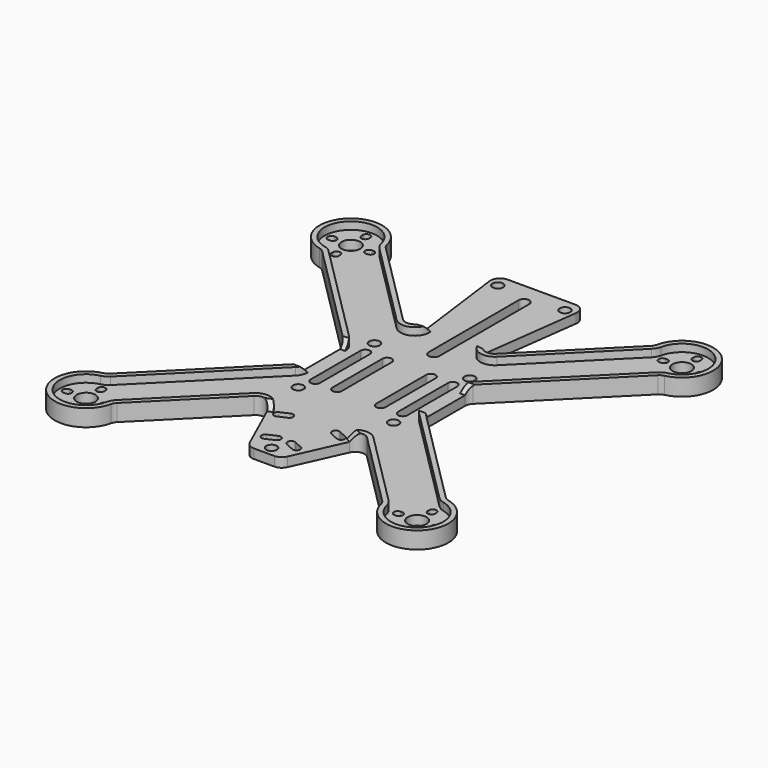
from build123d import *

# Parameters (mm, degrees)
F0_R     = 3
F0_R_2   = 1.7
F1_DEPTH = 3
F2_DEPTH = 5.4
F3_SIZE  = 2.39999


# Not quite as in the source:
# - a fillet or chamfer is up to 0.001 mm smaller than in the source, because OpenCascade refuses the exact size


with BuildPart() as f1:
    # F0 (on Top) → F1 (new body)
    with BuildSketch(Plane.XY):
        with BuildLine():
            Line((20, 0), (20, 7.4436508139))
            Line((20, 7.4436508139), (18.4, 7.4436508139))
            ThreePointArc((18.4, 7.4436508139), (18.7501541504, 9.2039946028), (19.7473088065, 10.6963420074))
            Line((19.7473088065, 10.6963420074), (52.626503914, 43.5755371148))
            ThreePointArc((52.626503914, 43.5755371148), (53.6562447149, 44.3500647573), (54.8604029925, 44.8086081338))
            ThreePointArc((54.8604029925, 44.8086081338), (58.939696962, 58.939696962), (44.8086081338, 54.8604029925))
            ThreePointArc((44.8086081338, 54.8604029925), (44.3500647573, 53.6562447149), (43.5755371148, 52.626503914))
            Line((43.5755371148, 52.626503914), (16.0551666535, 25.1061334527))
            ThreePointArc((16.0551666535, 25.1061334527), (10.770303635, 24.2320489467), (8.241146365, 28.9540362775))
            Line((8.241146365, 28.9540362775), (9.8276956154, 28.7470061448))
            Line((9.8276956154, 28.7470061448), (13.8552706772, 59.6118185013))
            ThreePointArc((13.8552706772, 59.6118185013), (13.1348803837, 61.9793250749), (10.8804908326, 63))
            Line((10.8804908326, 63), (0, 63))
            Line((0, 63), (-10.8804908326, 63))
            ThreePointArc((-10.8804908326, 63), (-13.1348803837, 61.9793250749), (-13.8552706772, 59.6118185013))
            Line((-13.8552706772, 59.6118185013), (-9.8276956154, 28.7470061448))
            Line((-9.8276956154, 28.7470061448), (-8.241146365, 28.9540362775))
            ThreePointArc((-8.241146365, 28.9540362775), (-10.770303635, 24.2320489467), (-16.0551666535, 25.1061334527))
            Line((-16.0551666535, 25.1061334527), (-43.5755371148, 52.626503914))
            ThreePointArc((-43.5755371148, 52.626503914), (-44.3500647573, 53.6562447149), (-44.8086081338, 54.8604029925))
            ThreePointArc((-44.8086081338, 54.8604029925), (-58.939696962, 58.939696962), (-54.8604029925, 44.8086081338))
            ThreePointArc((-54.8604029925, 44.8086081338), (-53.6562447149, 44.3500647573), (-52.626503914, 43.5755371148))
            Line((-52.626503914, 43.5755371148), (-19.7473088065, 10.6963420074))
            ThreePointArc((-19.7473088065, 10.6963420074), (-18.7501541504, 9.2039946028), (-18.4, 7.4436508139))
            Line((-18.4, 7.4436508139), (-20, 7.4436508139))
            Line((-20, 7.4436508139), (-20, 0))
            Line((-20, 0), (-20, -7.4436508139))
            Line((-20, -7.4436508139), (-18.4, -7.4436508139))
            ThreePointArc((-18.4, -7.4436508139), (-18.7501541504, -9.2039946028), (-19.7473088065, -10.6963420074))
            Line((-19.7473088065, -10.6963420074), (-52.626503914, -43.5755371148))
            ThreePointArc((-52.626503914, -43.5755371148), (-53.6562447149, -44.3500647573), (-54.8604029925, -44.8086081338))
            ThreePointArc((-54.8604029925, -44.8086081338), (-58.939696962, -58.939696962), (-44.8086081338, -54.8604029925))
            ThreePointArc((-44.8086081338, -54.8604029925), (-44.3500647573, -53.6562447149), (-43.5755371148, -52.626503914))
            Line((-43.5755371148, -52.626503914), (-19.2033018184, -28.2542686176))
            ThreePointArc((-19.2033018184, -28.2542686176), (-15.1223546276, -26.9821402563), (-11.7566370429, -29.6173604901))
            Line((-11.7566370429, -29.6173604901), (-13.2154104627, -30.2746124278))
            Line((-13.2154104627, -30.2746124278), (-6.025635767, -46.2323473832))
            ThreePointArc((-6.025635767, -46.2323473832), (-4.9187718494, -47.5196271698), (-3.2904356048, -48))
            Line((-3.2904356048, -48), (0, -48))
            Line((0, -48), (3.2904356048, -48))
            ThreePointArc((3.2904356048, -48), (4.9187718494, -47.5196271698), (6.025635767, -46.2323473832))
            Line((6.025635767, -46.2323473832), (13.2154104627, -30.2746124278))
            Line((13.2154104627, -30.2746124278), (11.7566370429, -29.6173604901))
            ThreePointArc((11.7566370429, -29.6173604901), (15.1223546276, -26.9821402563), (19.2033018184, -28.2542686176))
            Line((19.2033018184, -28.2542686176), (43.5755371148, -52.626503914))
            ThreePointArc((43.5755371148, -52.626503914), (44.3500647573, -53.6562447149), (44.8086081338, -54.8604029925))
            ThreePointArc((44.8086081338, -54.8604029925), (58.939696962, -58.939696962), (54.8604029925, -44.8086081338))
            ThreePointArc((54.8604029925, -44.8086081338), (53.6562447149, -44.3500647573), (52.626503914, -43.5755371148))
            Line((52.626503914, -43.5755371148), (19.7473088065, -10.6963420074))
            ThreePointArc((19.7473088065, -10.6963420074), (18.7501541504, -9.2039946028), (18.4, -7.4436508139))
            Line((18.4, -7.4436508139), (20, -7.4436508139))
            Line((20, -7.4436508139), (20, 0))
        make_face()
        with BuildLine():
            Line((-54.2, -59.25), (-54.2, -58.75))
            ThreePointArc((-54.2, -58.75), (-53, -57.55), (-51.8, -58.75))
            Line((-51.8, -58.75), (-51.8, -59.25))
            ThreePointArc((-51.8, -59.25), (-53, -60.45), (-54.2, -59.25))
        make_face(mode=Mode.SUBTRACT)
        with BuildLine():
            Line((-59.25, -51.8), (-58.75, -51.8))
            ThreePointArc((-58.75, -51.8), (-57.55, -53), (-58.75, -54.2))
            Line((-58.75, -54.2), (-59.25, -54.2))
            ThreePointArc((-59.25, -54.2), (-60.45, -53), (-59.25, -51.8))
        make_face(mode=Mode.SUBTRACT)
        with Locations((-53, -53)):
            Circle(F0_R, mode=Mode.SUBTRACT)
        with BuildLine():
            Line((-46.75, -54.2), (-47.25, -54.2))
            ThreePointArc((-47.25, -54.2), (-48.45, -53), (-47.25, -51.8))
            Line((-47.25, -51.8), (-46.75, -51.8))
            ThreePointArc((-46.75, -51.8), (-45.55, -53), (-46.75, -54.2))
        make_face(mode=Mode.SUBTRACT)
        with BuildLine():
            Line((-51.8, -46.75), (-51.8, -47.25))
            ThreePointArc((-51.8, -47.25), (-53, -48.45), (-54.2, -47.25))
            Line((-54.2, -47.25), (-54.2, -46.75))
            ThreePointArc((-54.2, -46.75), (-53, -45.55), (-51.8, -46.75))
        make_face(mode=Mode.SUBTRACT)
        with BuildLine():
            ThreePointArc((-4.4950166018, -42.3264274481), (-6.0820356199, -41.7252863365), (-5.4808945083, -40.1382673183))
            Line((-5.4808945083, -40.1382673183), (-2.7456943461, -38.9059199351))
            ThreePointArc((-2.7456943461, -38.9059199351), (-1.158675328, -39.5070610467), (-1.7598164396, -41.0940800649))
            Line((-1.7598164396, -41.0940800649), (-4.4950166018, -42.3264274481))
        make_face(mode=Mode.SUBTRACT)
        with BuildLine():
            ThreePointArc((-9.629797365, -30.9297601057), (-11.2168163832, -30.3286189941), (-10.6156752716, -28.7415999759))
            Line((-10.6156752716, -28.7415999759), (-7.8804751094, -27.5092525927))
            ThreePointArc((-7.8804751094, -27.5092525927), (-6.2934560912, -28.1103937043), (-6.8945972028, -29.6974127225))
            Line((-6.8945972028, -29.6974127225), (-9.629797365, -30.9297601057))
        make_face(mode=Mode.SUBTRACT)
        with Locations((-15.25, -15.25)):
            Circle(F0_R_2, mode=Mode.SUBTRACT)
        with Locations((0, -45)):
            Circle(F0_R_2, mode=Mode.SUBTRACT)
        with BuildLine():
            Line((2.7456943461, -38.9059199351), (5.4808945083, -40.1382673183))
            ThreePointArc((5.4808945083, -40.1382673183), (6.0820356199, -41.7252863365), (4.4950166018, -42.3264274481))
            Line((4.4950166018, -42.3264274481), (1.7598164396, -41.0940800649))
            ThreePointArc((1.7598164396, -41.0940800649), (1.158675328, -39.5070610467), (2.7456943461, -38.9059199351))
        make_face(mode=Mode.SUBTRACT)
        with BuildLine():
            ThreePointArc((47.25, -51.8), (48.45, -53), (47.25, -54.2))
            Line((47.25, -54.2), (46.75, -54.2))
            ThreePointArc((46.75, -54.2), (45.55, -53), (46.75, -51.8))
            Line((46.75, -51.8), (47.25, -51.8))
        make_face(mode=Mode.SUBTRACT)
        with BuildLine():
            ThreePointArc((54.2, -59.25), (53, -60.45), (51.8, -59.25))
            Line((51.8, -59.25), (51.8, -58.75))
            ThreePointArc((51.8, -58.75), (53, -57.55), (54.2, -58.75))
            Line((54.2, -58.75), (54.2, -59.25))
        make_face(mode=Mode.SUBTRACT)
        with Locations((53, -53)):
            Circle(F0_R, mode=Mode.SUBTRACT)
        with BuildLine():
            ThreePointArc((58.75, -54.2), (57.55, -53), (58.75, -51.8))
            Line((58.75, -51.8), (59.25, -51.8))
            ThreePointArc((59.25, -51.8), (60.45, -53), (59.25, -54.2))
            Line((59.25, -54.2), (58.75, -54.2))
        make_face(mode=Mode.SUBTRACT)
        with BuildLine():
            ThreePointArc((54.2, -47.25), (53, -48.45), (51.8, -47.25))
            Line((51.8, -47.25), (51.8, -46.75))
            ThreePointArc((51.8, -46.75), (53, -45.55), (54.2, -46.75))
            Line((54.2, -46.75), (54.2, -47.25))
        make_face(mode=Mode.SUBTRACT)
        with BuildLine():
            Line((7.8804751094, -27.5092525927), (10.6156752716, -28.7415999759))
            ThreePointArc((10.6156752716, -28.7415999759), (11.2168163832, -30.3286189941), (9.629797365, -30.9297601057))
            Line((9.629797365, -30.9297601057), (6.8945972028, -29.6974127225))
            ThreePointArc((6.8945972028, -29.6974127225), (6.2934560912, -28.1103937043), (7.8804751094, -27.5092525927))
        make_face(mode=Mode.SUBTRACT)
        with Locations((15.25, -15.25)):
            Circle(F0_R_2, mode=Mode.SUBTRACT)
        with BuildLine():
            ThreePointArc((-15.5, 10), (-14, 11.5), (-12.5, 10))
            Line((-12.5, 10), (-12.5, 0))
            Line((-12.5, 0), (-12.5, -10))
            ThreePointArc((-12.5, -10), (-14, -11.5), (-15.5, -10))
            Line((-15.5, -10), (-15.5, 0))
            Line((-15.5, 0), (-15.5, 10))
        make_face(mode=Mode.SUBTRACT)
        with BuildLine():
            Line((-5.5, 10), (-5.5, 0))
            Line((-5.5, 0), (-5.5, -10))
            ThreePointArc((-5.5, -10), (-7, -11.5), (-8.5, -10))
            Line((-8.5, -10), (-8.5, 0))
            Line((-8.5, 0), (-8.5, 10))
            ThreePointArc((-8.5, 10), (-7, 11.5), (-5.5, 10))
        make_face(mode=Mode.SUBTRACT)
        with Locations((-15.25, 15.25)):
            Circle(F0_R_2, mode=Mode.SUBTRACT)
        with BuildLine():
            ThreePointArc((-54.2, 47.25), (-53, 48.45), (-51.8, 47.25))
            Line((-51.8, 47.25), (-51.8, 46.75))
            ThreePointArc((-51.8, 46.75), (-53, 45.55), (-54.2, 46.75))
            Line((-54.2, 46.75), (-54.2, 47.25))
        make_face(mode=Mode.SUBTRACT)
        with BuildLine():
            ThreePointArc((-58.75, 54.2), (-57.55, 53), (-58.75, 51.8))
            Line((-58.75, 51.8), (-59.25, 51.8))
            ThreePointArc((-59.25, 51.8), (-60.45, 53), (-59.25, 54.2))
            Line((-59.25, 54.2), (-58.75, 54.2))
        make_face(mode=Mode.SUBTRACT)
        with Locations((-53, 53)):
            Circle(F0_R, mode=Mode.SUBTRACT)
        with BuildLine():
            Line((-51.8, 59.25), (-51.8, 58.75))
            ThreePointArc((-51.8, 58.75), (-53, 57.55), (-54.2, 58.75))
            Line((-54.2, 58.75), (-54.2, 59.25))
            ThreePointArc((-54.2, 59.25), (-53, 60.45), (-51.8, 59.25))
        make_face(mode=Mode.SUBTRACT)
        with BuildLine():
            ThreePointArc((-47.25, 51.8), (-48.45, 53), (-47.25, 54.2))
            Line((-47.25, 54.2), (-46.75, 54.2))
            ThreePointArc((-46.75, 54.2), (-45.55, 53), (-46.75, 51.8))
            Line((-46.75, 51.8), (-47.25, 51.8))
        make_face(mode=Mode.SUBTRACT)
        with Locations((-10.75, 59)):
            Circle(F0_R_2, mode=Mode.SUBTRACT)
        with BuildLine():
            Line((5.5, 0), (5.5, 10))
            ThreePointArc((5.5, 10), (7, 11.5), (8.5, 10))
            Line((8.5, 10), (8.5, 0))
            Line((8.5, 0), (8.5, -10))
            ThreePointArc((8.5, -10), (7, -11.5), (5.5, -10))
            Line((5.5, -10), (5.5, 0))
        make_face(mode=Mode.SUBTRACT)
        with BuildLine():
            Line((12.5, 0), (12.5, 10))
            ThreePointArc((12.5, 10), (14, 11.5), (15.5, 10))
            Line((15.5, 10), (15.5, 0))
            Line((15.5, 0), (15.5, -10))
            ThreePointArc((15.5, -10), (14, -11.5), (12.5, -10))
            Line((12.5, -10), (12.5, 0))
        make_face(mode=Mode.SUBTRACT)
        with Locations((15.25, 15.25)):
            Circle(F0_R_2, mode=Mode.SUBTRACT)
        with BuildLine():
            Line((1.7, 56), (1.7, 20))
            ThreePointArc((1.7, 20), (0, 18.3), (-1.7, 20))
            Line((-1.7, 20), (-1.7, 56))
            ThreePointArc((-1.7, 56), (0, 57.7), (1.7, 56))
        make_face(mode=Mode.SUBTRACT)
        with Locations((10.75, 59)):
            Circle(F0_R_2, mode=Mode.SUBTRACT)
        with BuildLine():
            Line((51.8, 46.75), (51.8, 47.25))
            ThreePointArc((51.8, 47.25), (53, 48.45), (54.2, 47.25))
            Line((54.2, 47.25), (54.2, 46.75))
            ThreePointArc((54.2, 46.75), (53, 45.55), (51.8, 46.75))
        make_face(mode=Mode.SUBTRACT)
        with BuildLine():
            Line((46.75, 54.2), (47.25, 54.2))
            ThreePointArc((47.25, 54.2), (48.45, 53), (47.25, 51.8))
            Line((47.25, 51.8), (46.75, 51.8))
            ThreePointArc((46.75, 51.8), (45.55, 53), (46.75, 54.2))
        make_face(mode=Mode.SUBTRACT)
        with Locations((53, 53)):
            Circle(F0_R, mode=Mode.SUBTRACT)
        with BuildLine():
            Line((59.25, 51.8), (58.75, 51.8))
            ThreePointArc((58.75, 51.8), (57.55, 53), (58.75, 54.2))
            Line((58.75, 54.2), (59.25, 54.2))
            ThreePointArc((59.25, 54.2), (60.45, 53), (59.25, 51.8))
        make_face(mode=Mode.SUBTRACT)
        with BuildLine():
            Line((54.2, 59.25), (54.2, 58.75))
            ThreePointArc((54.2, 58.75), (53, 57.55), (51.8, 58.75))
            Line((51.8, 58.75), (51.8, 59.25))
            ThreePointArc((51.8, 59.25), (53, 60.45), (54.2, 59.25))
        make_face(mode=Mode.SUBTRACT)
    extrude(amount=F1_DEPTH)

    # F0 (on Top) → F2 (join)
    with BuildSketch(Plane.XY):
        with BuildLine():
            Line((-8.241146365, 28.9540362775), (-9.8276956154, 28.7470061448))
            ThreePointArc((-9.8276956154, 28.7470061448), (-11.4771460089, 25.66744919), (-14.9237958036, 26.2375043026))
            Line((-14.9237958036, 26.2375043026), (-42.4441662649, 53.7578747639))
            ThreePointArc((-42.4441662649, 53.7578747639), (-42.9492929883, 54.4294448514), (-43.2483430164, 55.2147654673))
            ThreePointArc((-43.2483430164, 55.2147654673), (-60.0710678119, 60.0710678119), (-55.2147654673, 43.2483430164))
            ThreePointArc((-55.2147654673, 43.2483430164), (-54.4294448514, 42.9492929883), (-53.7578747639, 42.4441662649))
            Line((-53.7578747639, 42.4441662649), (-20.8786796564, 9.5649711575))
            ThreePointArc((-20.8786796564, 9.5649711575), (-20.2283614025, 8.591701111), (-20, 7.4436508139))
            Line((-20, 7.4436508139), (-18.4, 7.4436508139))
            ThreePointArc((-18.4, 7.4436508139), (-18.7501541504, 9.2039946028), (-19.7473088065, 10.6963420074))
            Line((-19.7473088065, 10.6963420074), (-52.626503914, 43.5755371148))
            ThreePointArc((-52.626503914, 43.5755371148), (-53.6562447149, 44.3500647573), (-54.8604029925, 44.8086081338))
            ThreePointArc((-54.8604029925, 44.8086081338), (-58.939696962, 58.939696962), (-44.8086081338, 54.8604029925))
            ThreePointArc((-44.8086081338, 54.8604029925), (-44.3500647573, 53.6562447149), (-43.5755371148, 52.626503914))
            Line((-43.5755371148, 52.626503914), (-16.0551666535, 25.1061334527))
            ThreePointArc((-16.0551666535, 25.1061334527), (-10.770303635, 24.2320489467), (-8.241146365, 28.9540362775))
        make_face()
        with BuildLine():
            ThreePointArc((53.7578747639, 42.4441662649), (54.4294448514, 42.9492929883), (55.2147654673, 43.2483430164))
            ThreePointArc((55.2147654673, 43.2483430164), (60.0710678119, 60.0710678119), (43.2483430164, 55.2147654673))
            ThreePointArc((43.2483430164, 55.2147654673), (42.9492929883, 54.4294448514), (42.4441662649, 53.7578747639))
            Line((42.4441662649, 53.7578747639), (14.9237958036, 26.2375043026))
            ThreePointArc((14.9237958036, 26.2375043026), (11.4771460089, 25.66744919), (9.8276956154, 28.7470061448))
            Line((9.8276956154, 28.7470061448), (8.241146365, 28.9540362775))
            ThreePointArc((8.241146365, 28.9540362775), (10.770303635, 24.2320489467), (16.0551666535, 25.1061334527))
            Line((16.0551666535, 25.1061334527), (43.5755371148, 52.626503914))
            ThreePointArc((43.5755371148, 52.626503914), (44.3500647573, 53.6562447149), (44.8086081338, 54.8604029925))
            ThreePointArc((44.8086081338, 54.8604029925), (58.939696962, 58.939696962), (54.8604029925, 44.8086081338))
            ThreePointArc((54.8604029925, 44.8086081338), (53.6562447149, 44.3500647573), (52.626503914, 43.5755371148))
            Line((52.626503914, 43.5755371148), (19.7473088065, 10.6963420074))
            ThreePointArc((19.7473088065, 10.6963420074), (18.7501541504, 9.2039946028), (18.4, 7.4436508139))
            Line((18.4, 7.4436508139), (20, 7.4436508139))
            ThreePointArc((20, 7.4436508139), (20.2283614025, 8.591701111), (20.8786796564, 9.5649711575))
            Line((20.8786796564, 9.5649711575), (53.7578747639, 42.4441662649))
        make_face()
        with BuildLine():
            ThreePointArc((20.8786796564, -9.5649711575), (20.2283614025, -8.591701111), (20, -7.4436508139))
            Line((20, -7.4436508139), (18.4, -7.4436508139))
            ThreePointArc((18.4, -7.4436508139), (18.7501541504, -9.2039946028), (19.7473088065, -10.6963420074))
            Line((19.7473088065, -10.6963420074), (52.626503914, -43.5755371148))
            ThreePointArc((52.626503914, -43.5755371148), (53.6562447149, -44.3500647573), (54.8604029925, -44.8086081338))
            ThreePointArc((54.8604029925, -44.8086081338), (58.939696962, -58.939696962), (44.8086081338, -54.8604029925))
            ThreePointArc((44.8086081338, -54.8604029925), (44.3500647573, -53.6562447149), (43.5755371148, -52.626503914))
            Line((43.5755371148, -52.626503914), (19.2033018184, -28.2542686176))
            ThreePointArc((19.2033018184, -28.2542686176), (15.1223546276, -26.9821402563), (11.7566370429, -29.6173604901))
            Line((11.7566370429, -29.6173604901), (13.2154104627, -30.2746124278))
            ThreePointArc((13.2154104627, -30.2746124278), (15.4104436702, -28.5559905362), (18.0719309685, -29.3856394675))
            Line((18.0719309685, -29.3856394675), (42.4441662649, -53.7578747639))
            ThreePointArc((42.4441662649, -53.7578747639), (42.9492929883, -54.4294448514), (43.2483430164, -55.2147654673))
            ThreePointArc((43.2483430164, -55.2147654673), (60.0710678119, -60.0710678119), (55.2147654673, -43.2483430164))
            ThreePointArc((55.2147654673, -43.2483430164), (54.4294448514, -42.9492929883), (53.7578747639, -42.4441662649))
            Line((53.7578747639, -42.4441662649), (20.8786796564, -9.5649711575))
        make_face()
        with BuildLine():
            ThreePointArc((-18.0719309685, -29.3856394675), (-15.4104436702, -28.5559905362), (-13.2154104627, -30.2746124278))
            Line((-13.2154104627, -30.2746124278), (-11.7566370429, -29.6173604901))
            ThreePointArc((-11.7566370429, -29.6173604901), (-15.1223546276, -26.9821402563), (-19.2033018184, -28.2542686176))
            Line((-19.2033018184, -28.2542686176), (-43.5755371148, -52.626503914))
            ThreePointArc((-43.5755371148, -52.626503914), (-44.3500647573, -53.6562447149), (-44.8086081338, -54.8604029925))
            ThreePointArc((-44.8086081338, -54.8604029925), (-58.939696962, -58.939696962), (-54.8604029925, -44.8086081338))
            ThreePointArc((-54.8604029925, -44.8086081338), (-53.6562447149, -44.3500647573), (-52.626503914, -43.5755371148))
            Line((-52.626503914, -43.5755371148), (-19.7473088065, -10.6963420074))
            ThreePointArc((-19.7473088065, -10.6963420074), (-18.7501541504, -9.2039946028), (-18.4, -7.4436508139))
            Line((-18.4, -7.4436508139), (-20, -7.4436508139))
            ThreePointArc((-20, -7.4436508139), (-20.2283614025, -8.591701111), (-20.8786796564, -9.5649711575))
            Line((-20.8786796564, -9.5649711575), (-53.7578747639, -42.4441662649))
            ThreePointArc((-53.7578747639, -42.4441662649), (-54.4294448514, -42.9492929883), (-55.2147654673, -43.2483430164))
            ThreePointArc((-55.2147654673, -43.2483430164), (-60.0710678119, -60.0710678119), (-43.2483430164, -55.2147654673))
            ThreePointArc((-43.2483430164, -55.2147654673), (-42.9492929883, -54.4294448514), (-42.4441662649, -53.7578747639))
            Line((-42.4441662649, -53.7578747639), (-18.0719309685, -29.3856394675))
        make_face()
    extrude(amount=F2_DEPTH)

    # F3 (size 2.4 in the source; OpenCascade refuses exactly that, so slightly less here)
    f3_edges = [f1.edges().sort_by_distance(p)[0] for p in [
        (-9.034421, 28.850521, 5.4),
        (-19.2, 7.443651, 5.4),
        (-19.2, -7.443651, 5.4),
        (19.2, -7.443651, 5.4),
        (19.2, 7.443651, 5.4),
        (9.034421, 28.850521, 5.4),
        (12.486024, -29.945986, 5.4),
        (-12.486024, -29.945986, 5.4),
    ]]
    chamfer(f3_edges, length=F3_SIZE)


solid = f1.part
